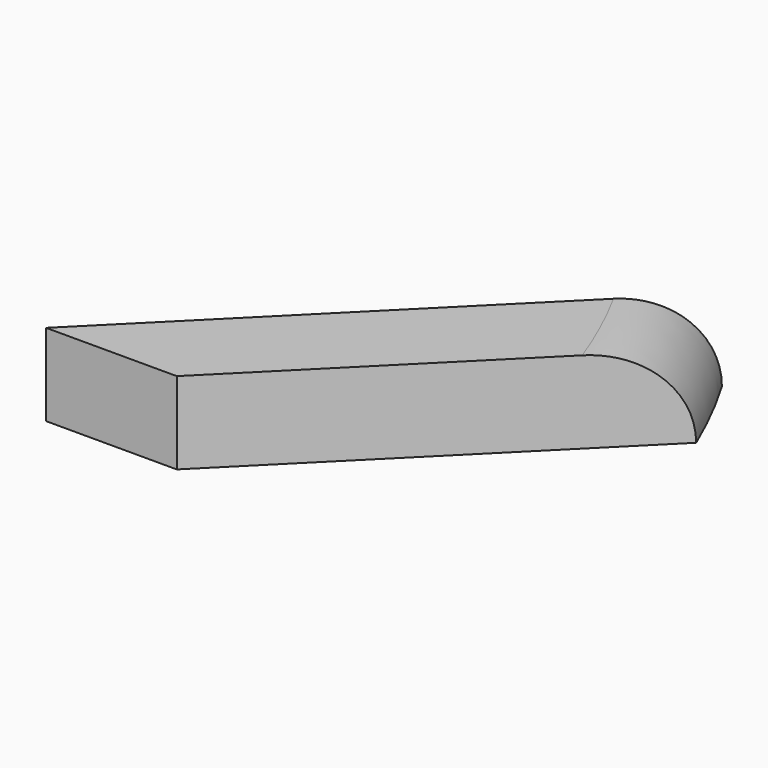
from build123d import *

# Parameters (mm, degrees)
F2_DEPTH = 25.4
F3_R     = 25.39999


# Not quite as in the source:
# - a fillet or chamfer is up to 0.001 mm smaller than in the source, because OpenCascade refuses the exact size


with BuildPart() as f2:
    # F1 (on face) → F2 (new body)
    with BuildSketch(Plane.XY):
        with BuildLine():
            Line((196.9228733519, 116.1005682623), (80.8223050896, 0))
            Line((80.8223050896, 0), (121.2334576344, 0))
            Line((121.2334576344, 0), (210.4652929995, 89.2318353651))
            ThreePointArc((210.4652929995, 89.2318353651), (204.1366251379, 102.889252487), (196.9228733519, 116.1005682623))
        make_face()
    extrude(amount=F2_DEPTH)

    # F3 (radius 25.4 in the source; OpenCascade refuses exactly that, so slightly less here)
    f3_edges = [f2.edges().sort_by_distance(p)[0] for p in [
        (204.136625, 102.889252, 25.4),
    ]]
    fillet(f3_edges, radius=F3_R)


solid = f2.part
